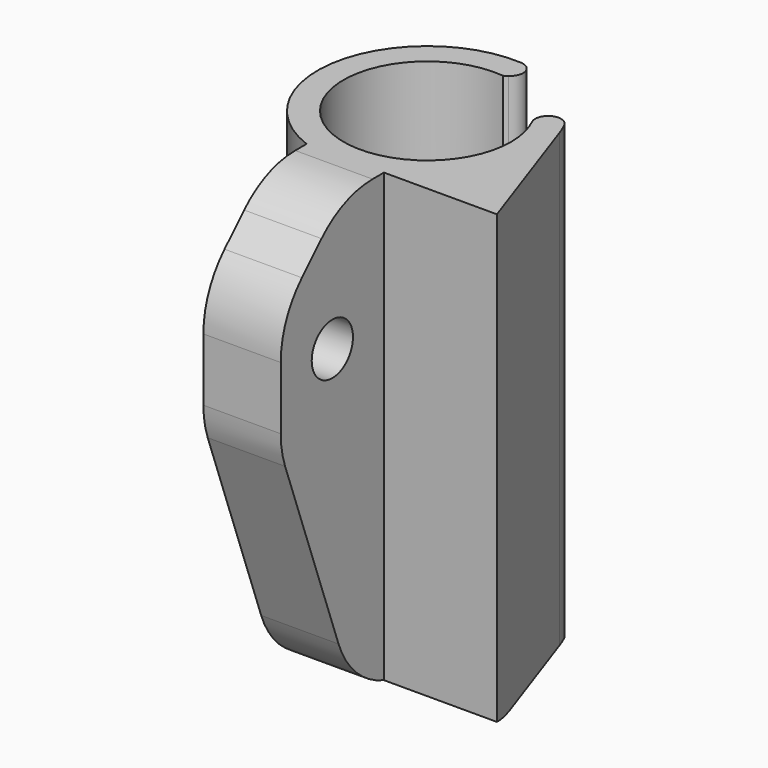
from build123d import *

# Parameters (mm, degrees)
F1_DEPTH      = 15
F1_DEPTH_BACK = 20
F2_R          = 2
F3_DEPTH      = 14.7596476454
F4_R          = 0.99999
F5_SIZE2      = 7.2794046853
F5_SIZE       = 20
F6_SIZE       = 6
F7_T1_DEPTH   = 20.4974746831
F7_T3_DEPTH   = 30.5072638373
F7_T5_DEPTH   = 12.1714443248


# Not quite as in the source:
# - a fillet or chamfer that OpenCascade refuses, or shapes differently, is made with other operations: its cross-section is extruded or revolved along the edge and cut away or added
# - a fillet or chamfer is up to 0.001 mm smaller than in the source, because OpenCascade refuses the exact size
# - a feature names something its author has since deleted; it is built from what else it names


with BuildPart() as f1:
    # F0 (on Top) → F1 (new body, two sides)
    with BuildSketch(Plane.XY) as f1_sk:
        with BuildLine():
            Line((0, 10), (0, 0))
            Line((0, 0), (6, 0))
            Line((6, 0), (6, 10))
            ThreePointArc((6, 10), (3, 9.4529868603), (0, 10))
        make_face()
        with BuildLine():
            ThreePointArc((11.5, 17.9529868603), (9.9910657271, 13.1182169588), (6, 10))
            Line((6, 10), (14.7586476454, 10))
            Line((14.7586476454, 10), (11.0298702995, 20.7406710197))
            ThreePointArc((11.0298702995, 20.7406710197), (11.3816435604, 19.3665112594), (11.5, 17.9529868603))
        make_face()
        with BuildLine():
            ThreePointArc((5.9635743738, 25.9196189549), (-4.9598303138, 20.9347818526), (0, 10))
            ThreePointArc((0, 10), (3, 9.4529868603), (6, 10))
            ThreePointArc((6, 10), (9.9910657271, 13.1182169588), (11.5, 17.9529868603))
            ThreePointArc((11.5, 17.9529868603), (11.3816435604, 19.3665112594), (11.0298702995, 20.7406710197))
            ThreePointArc((11.0298702995, 20.7406710197), (10.6165760284, 21.7262837746), (10.0828666254, 22.6522421594))
            Line((10.0828666254, 22.6522421594), (8.4163097724, 21.5465350302))
            ThreePointArc((8.4163097724, 21.5465350302), (9.2231830087, 19.8296842892), (9.5, 17.9529868603))
            ThreePointArc((9.5, 17.9529868603), (-1.83621149, 13.6100548526), (3.6965974081, 24.4155522991))
            Line((3.6965974081, 24.4155522991), (5.9635743738, 25.9196189549))
        make_face()
    extrude(amount=F1_DEPTH)
    extrude(f1_sk.sketch, amount=-F1_DEPTH_BACK)

    # F2 (on face) → F3 (cut, through all)
    with BuildSketch(Plane(origin=(0, 0, 0), x_dir=(0, -1, 0), z_dir=(-1, 0, 0))):
        with Locations((-5, 5)):
            Circle(F2_R)
    extrude(amount=-F3_DEPTH, mode=Mode.SUBTRACT)

    # F4 (radius 1 in the source; OpenCascade refuses exactly that, so slightly less here)
    f4_edges = [f1.edges().sort_by_distance(p)[0] for p in [
        (5.963574, 25.919619, -2.5),
        (8.41631, 21.546535, -2.5),
        (10.082867, 22.652242, -2.5),
    ]]
    fillet(f4_edges, radius=F4_R)

    # F5
    f5_edges = [f1.edges().sort_by_distance(p)[0] for p in [
        (3, 0, -20),
    ]]
    f5_side = f1.faces().sort_by_distance((3, 0, -2.5))[0]
    chamfer(f5_edges, length=F5_SIZE, length2=F5_SIZE2, reference=f5_side)

    # F6
    f6_edges = [f1.edges().sort_by_distance(p)[0] for p in [
        (3, 0, 15),
    ]]
    chamfer(f6_edges, length=F6_SIZE)

    # F7: fillet of radius 7 on 4 edges, made by hand

    # F7_s2 → F7_t1 (cut)
    with BuildSketch(Plane.YZ.offset(-7.2487373415)):
        with BuildLine():
            ThreePointArc((0, 6.1005050634), (0.5328432724, 8.7792890899), (2.0502525317, 11.0502525317))
            Line((2.0502525317, 11.0502525317), (0, 9))
            Line((0, 9), (0, 6.1005050634))
        make_face()
        with BuildLine():
            ThreePointArc((3.9497474683, 12.9497474683), (6.2207109101, 14.4671567276), (8.8994949366, 15))
            Line((8.8994949366, 15), (6, 15))
            Line((6, 15), (3.9497474683, 12.9497474683))
        make_face()
    extrude(amount=F7_T1_DEPTH, mode=Mode.SUBTRACT)

    # F7_s4 → F7_t3 (cut)
    with BuildSketch(Plane.YZ.offset(-12.2536319187)):
        with BuildLine():
            ThreePointArc((5.6030091073, -15.3941410033), (8.1658223983, -18.73406431), (12.1808574528, -20))
            Line((12.1808574528, -20), (7.2794046853, -20))
            Line((7.2794046853, -20), (5.6030091073, -15.3941410033))
        make_face()
    extrude(amount=F7_T3_DEPTH, mode=Mode.SUBTRACT)

    # F7_s6 → F7_t5 (cut)
    with BuildSketch(Plane.YZ.offset(-3.0857221624)):
        with BuildLine():
            ThreePointArc((0, 1.234288865), (0.1063457289, 0.0187516213), (0.4221516545, -1.1598521383))
            Line((0.4221516545, -1.1598521383), (0, 0))
            Line((0, 0), (0, 1.234288865))
        make_face()
    extrude(amount=F7_T5_DEPTH, mode=Mode.SUBTRACT)


solid = f1.part
